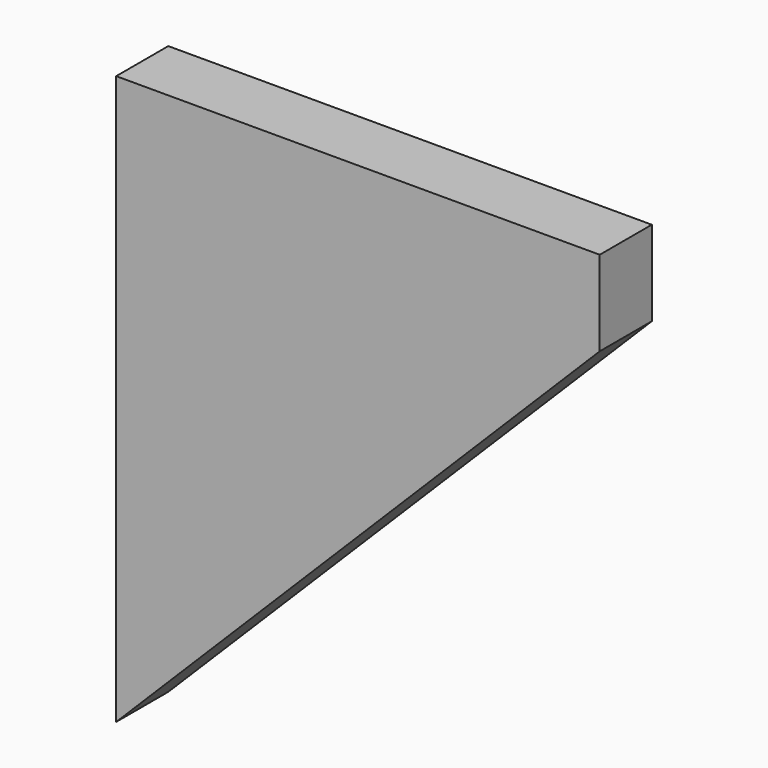
from build123d import *

# Parameters (mm, degrees)
F0_W        = 9.4349011779
F0_H        = 11.8184201419
F1_DEPTH    = 1.27
F2_T1_DEPTH = 53.5265983155


# Not quite as in the source:
# - a fillet or chamfer that OpenCascade refuses, or shapes differently, is made with other operations: its cross-section is extruded or revolved along the edge and cut away or added


with BuildPart() as f1:
    # F0 (on Front) → F1 (new body)
    with BuildSketch(Plane.XZ):
        with Locations((-34.5215313137, 36.3493505865)):
            Rectangle(F0_W, F0_H)
    extrude(amount=F1_DEPTH)

    # F2: chamfer of 10.16 on 1 edges, made by hand

    # F2_s2 → F2_t1 (cut)
    with BuildSketch(Plane.XZ.offset(-26.1282991577)):
        Polygon((-39.9640807247, 30.4401405156), (-29.8040807247, 40.6001405156), (-29.8040807247, 30.4401405156), align=None)
    extrude(amount=F2_T1_DEPTH, mode=Mode.SUBTRACT)


solid = f1.part
